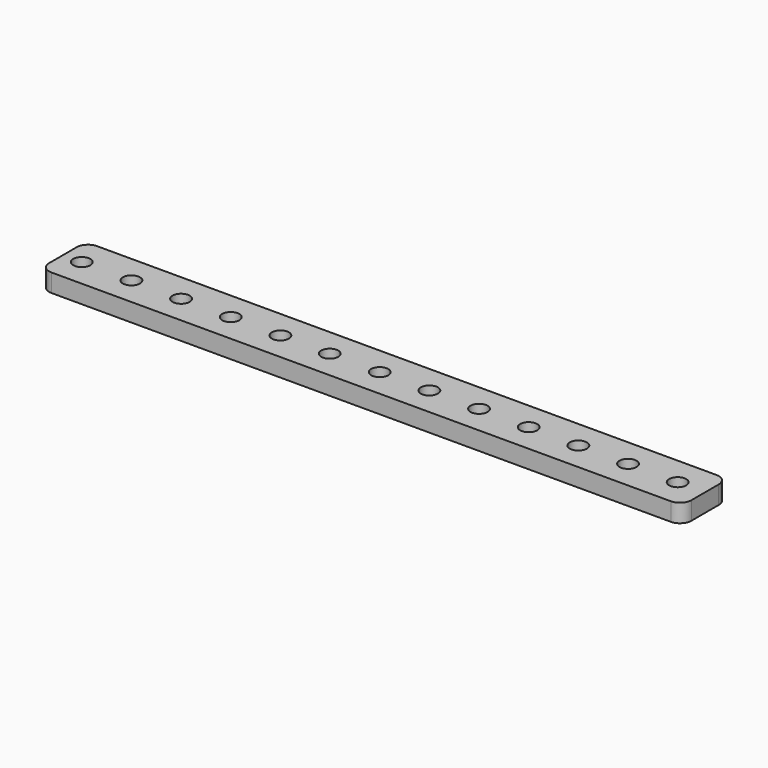
from build123d import *

# Parameters (mm, degrees)
F0_W     = 112.6090909091
F0_H     = 10
F0_R     = 1.5
F1_DEPTH = 3.175
F2_R     = 2


# Not quite as in the source:
# - a length typed as a fraction of an inch, garbled in the dataset ("3 / 203.2 mm" for 3/8 in), is restored


with BuildPart() as f1:
    # F0 (on Top) → F1 (new body)
    with BuildSketch(Plane.XY):
        with Locations((9.4590909091, 0)):
            Rectangle(F0_W, F0_H)
        with Locations((-43.5454545455, 0)):
            Circle(F0_R, mode=Mode.SUBTRACT)
        with Locations((-34.8363636364, 0)):
            Circle(F0_R, mode=Mode.SUBTRACT)
        with Locations((-26.1272727273, 0)):
            Circle(F0_R, mode=Mode.SUBTRACT)
        with Locations((-17.4181818182, 0)):
            Circle(F0_R, mode=Mode.SUBTRACT)
        with Locations((-8.7090909091, 0)):
            Circle(F0_R, mode=Mode.SUBTRACT)
        with Locations((-0.0571461482, 0)):
            Circle(F0_R, mode=Mode.SUBTRACT)
        with Locations((8.7090909091, 0)):
            Circle(F0_R, mode=Mode.SUBTRACT)
        with Locations((17.4181818182, 0)):
            Circle(F0_R, mode=Mode.SUBTRACT)
        with Locations((26.1272727273, 0)):
            Circle(F0_R, mode=Mode.SUBTRACT)
        with Locations((34.8363636364, 0)):
            Circle(F0_R, mode=Mode.SUBTRACT)
        with Locations((43.5454545455, 0)):
            Circle(F0_R, mode=Mode.SUBTRACT)
        with Locations((52.2545454545, 0)):
            Circle(F0_R, mode=Mode.SUBTRACT)
        with Locations((60.9636363636, 0)):
            Circle(F0_R, mode=Mode.SUBTRACT)
    extrude(amount=F1_DEPTH)

    # F2
    f2_edges = [f1.edges().sort_by_distance(p)[0] for p in [
        (-46.845455, 5, 1.5875),
        (-46.845455, -5, 1.5875),
        (65.763636, 5, 1.5875),
        (65.763636, -5, 1.5875),
    ]]
    fillet(f2_edges, radius=F2_R)


solid = f1.part
